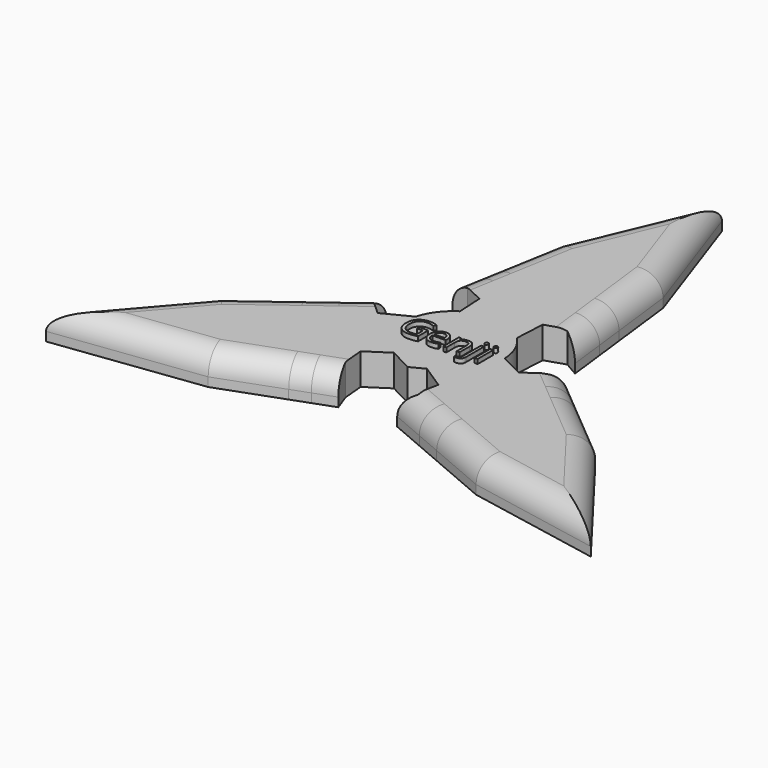
from build123d import *

# Parameters (mm, degrees)
F1_DEPTH     = 7
F2_R         = 5
F3_TEXT_SIZE = 8.0615537526
F4_DEPTH     = 1


# Not quite as in the source:
# - Text() gives the source's letters only with a copy of the font that has no kerning and outlines rounded to 1/6400 em; it was checked with that copy


with BuildPart() as f1:
    # F0 (on Top) → F1 (new body)
    with BuildSketch(Plane.XY):
        with BuildLine():
            ThreePointArc((5.1980970801, -9.9206747122), (9.5827628401, -5.7974698232), (11.2, 0))
            ThreePointArc((11.2, 0), (11.1976509695, 0.2293747246), (11.1906048635, 0.4586532334))
            Line((11.1906048635, 0.4586532334), (8.0356504368, 7.8018153052))
            ThreePointArc((8.0356504368, 7.8018153052), (1.3163126947, 11.1223792819), (-5.9925077834, 9.4620214788))
            ThreePointArc((-5.9925077834, 9.4620214788), (-6.7286502341, 8.9535057953), (-7.4218538812, 8.3878534182))
            Line((-7.4218538812, 8.3878534182), (-10.7743954684, 3.0581697616))
            ThreePointArc((-10.7743954684, 3.0581697616), (-10.290419356, -4.421229408), (-5.1980970801, -9.9206747122))
            ThreePointArc((-5.1980970801, -9.9206747122), (-1.3163126947, -11.1223792819), (2.7387450316, -10.8599850668))
            ThreePointArc((2.7387450316, -10.8599850668), (3.9961158219, -10.4628417907), (5.1980970801, -9.9206747122))
        make_face()
        with BuildLine():
            ThreePointArc((11.1906048635, 0.4586532334), (11.1976509695, 0.2293747246), (11.2, 0))
            ThreePointArc((11.2, 0), (9.5827628401, -5.7974698232), (5.1980970801, -9.9206747122))
            Line((5.1980970801, -9.9206747122), (3.0363366012, -11.053363885))
            Line((3.0363366012, -11.053363885), (8.3903111517, -14.5324452061))
            Line((8.3903111517, -14.5324452061), (7.4478763008, -19.0164396847))
            Line((7.4478763008, -19.0164396847), (4.2604654155, -20.8566922174))
            Line((4.2604654155, -20.8566922174), (11.7370859302, -24.0546467051))
            Line((11.7370859302, -24.0546467051), (25.603668997, -18.95442529))
            Line((25.603668997, -18.95442529), (26.6218720817, 0.3686850477))
            Line((26.6218720817, 0.3686850477), (22.8139994853, 3.5596574961))
            Line((22.8139994853, 3.5596574961), (20.2907988469, 0.5486548248))
            Line((20.2907988469, 0.5486548248), (16.4055937609, -2.1755951247))
            Line((16.4055937609, -2.1755951247), (11.1906048635, 0.4586532334))
        make_face()
        with BuildLine():
            Line((8.0356504368, 7.8018153052), (11.1906048635, 0.4586532334))
            ThreePointArc((11.1906048635, 0.4586532334), (10.290419356, 4.421229408), (8.0356504368, 7.8018153052))
        make_face()
        with BuildLine():
            Line((3.0363366012, -11.053363885), (5.1980970801, -9.9206747122))
            ThreePointArc((5.1980970801, -9.9206747122), (3.9961158219, -10.4628417907), (2.7387450316, -10.8599850668))
            Line((2.7387450316, -10.8599850668), (3.0363366012, -11.053363885))
        make_face()
        with BuildLine():
            ThreePointArc((-5.9925077834, 9.4620214788), (1.3163126947, 11.1223792819), (8.0356504368, 7.8018153052))
            Line((8.0356504368, 7.8018153052), (8.3903111517, 14.5324452061))
            Line((8.3903111517, 14.5324452061), (12.7447817061, 15.9582699231))
            Line((12.7447817061, 15.9582699231), (15.9321925914, 14.1180173904))
            Line((15.9321925914, 14.1180173904), (14.9633921606, 22.1919379345))
            Line((14.9633921606, 22.1919379345), (3.6131793168, 31.6506404265))
            Line((3.6131793168, 31.6506404265), (-13.6302266581, 22.8708749952))
            Line((-13.6302266581, 22.8708749952), (-14.489753563, 17.9776743682))
            Line((-14.489753563, 17.9776743682), (-10.6205484397, 17.2980198521))
            Line((-10.6205484397, 17.2980198521), (-6.3186762341, 15.2954585235))
            Line((-6.3186762341, 15.2954585235), (-5.9925077834, 9.4620214788))
        make_face()
        with BuildLine():
            Line((3.0363366012, -11.053363885), (2.7387450316, -10.8599850668))
            ThreePointArc((2.7387450316, -10.8599850668), (-1.3163126947, -11.1223792819), (-5.1980970801, -9.9206747122))
            Line((-5.1980970801, -9.9206747122), (0, -12.6443012838))
            Line((0, -12.6443012838), (3.0363366012, -11.053363885))
        make_face()
        with BuildLine():
            Line((-10.0869175268, -13.1198633988), (-5.1980970801, -9.9206747122))
            ThreePointArc((-5.1980970801, -9.9206747122), (-10.290419356, -4.421229408), (-10.7743954684, 3.0581697616))
            Line((-10.7743954684, 3.0581697616), (-16.7806223035, 0))
            Line((-16.7806223035, 0), (-20.1926580069, 3.0581697616))
            Line((-20.1926580069, 3.0581697616), (-20.1926580069, 6.7386748269))
            Line((-20.1926580069, 6.7386748269), (-26.7004780908, 1.8627087706))
            Line((-26.7004780908, 1.8627087706), (-29.2168483138, -12.6962151365))
            Line((-29.2168483138, -12.6962151365), (-12.9916454236, -23.2395600429))
            Line((-12.9916454236, -23.2395600429), (-8.3242459223, -21.5373318642))
            Line((-8.3242459223, -21.5373318642), (-9.6702504072, -17.8466746769))
            Line((-9.6702504072, -17.8466746769), (-10.0869175268, -13.1198633988))
        make_face()
        with BuildLine():
            Line((-10.7743954684, 3.0581697616), (-7.4218538812, 8.3878534182))
            ThreePointArc((-7.4218538812, 8.3878534182), (-9.480361521, 5.963450799), (-10.7743954684, 3.0581697616))
        make_face()
        Polygon((29.7958199429, -2.2910625992), (26.6218720817, 0.3686850477), (25.603668997, -18.95442529), (11.7370859302, -24.0546467051), (17.6323589973, -26.5762157648), (55.101781317, -34.1392541535), align=None)
        Polygon((3.6131793168, 31.6506404265), (14.9633921606, 22.1919379345), (14.1994984902, 28.5581787027), (2.0145707047, 64.7891694911), (-12.9137915589, 26.9494682968), (-13.6302266581, 22.8708749952), align=None)
        Polygon((41.1397027161, -11.7971625202), (29.7958199429, -2.2910625992), (55.101781317, -34.1392541535), (17.6323589973, -26.5762157648), (31.004252579, -32.2957393123), (61.1856488306, -38.0613842263), align=None)
        Polygon((2.0145707047, 64.7891694911), (14.1994984902, 28.5581787027), (12.4668043889, 42.9983400149), (2.3693012279, 72.0190183475), (-10.353208923, 41.5266089164), (-12.9137915589, 26.9494682968), align=None)
        Polygon((-16.8820283841, -24.6584056975), (-12.9916454236, -23.2395600429), (-29.2168483138, -12.6962151365), (-26.7004780908, 1.8627087706), (-31.8318574874, -1.9819629379), (-57.1163520217, -30.6499153376), align=None)
        Polygon((-30.7864937931, -29.7294463962), (-16.8820283841, -24.6584056975), (-57.1163520217, -30.6499153376), (-31.8318574874, -1.9819629379), (-43.471056968, -10.7026007026), (-63.5549500585, -33.9576341212), align=None)
    extrude(amount=F1_DEPTH)

    # F2
    f2_edges = [f1.edges().sort_by_distance(p)[0] for p in [
        (-12.421481, 29.752142, 7),
        (-3.991954, 56.772814, 7),
        (14.199498, 28.558179, 7),
        (7.418053, 57.508679, 7),
        (-31.831857, -1.981963, 7),
        (-53.513004, -22.330117, 7),
        (17.632359, -26.576216, 7),
        (46.094951, -35.178562, 7),
        (31.976851, -4.118753, 7),
        (51.162676, -24.929273, 7),
        (-47.170722, -31.84354, 7),
        (-19.55537, -25.633389, 7),
    ]]
    fillet(f2_edges, radius=F2_R)

    # F3 (on face) → F4 (join)
    with BuildSketch(Plane.XY.offset(7)):
        with Locations((-9.8847826011, -4.1636209935)):
            Text('Genji', F3_TEXT_SIZE, font='Open Sans', text_align=(TextAlign.LEFT, TextAlign.BOTTOM))
    extrude(amount=F4_DEPTH)


solid = f1.part
